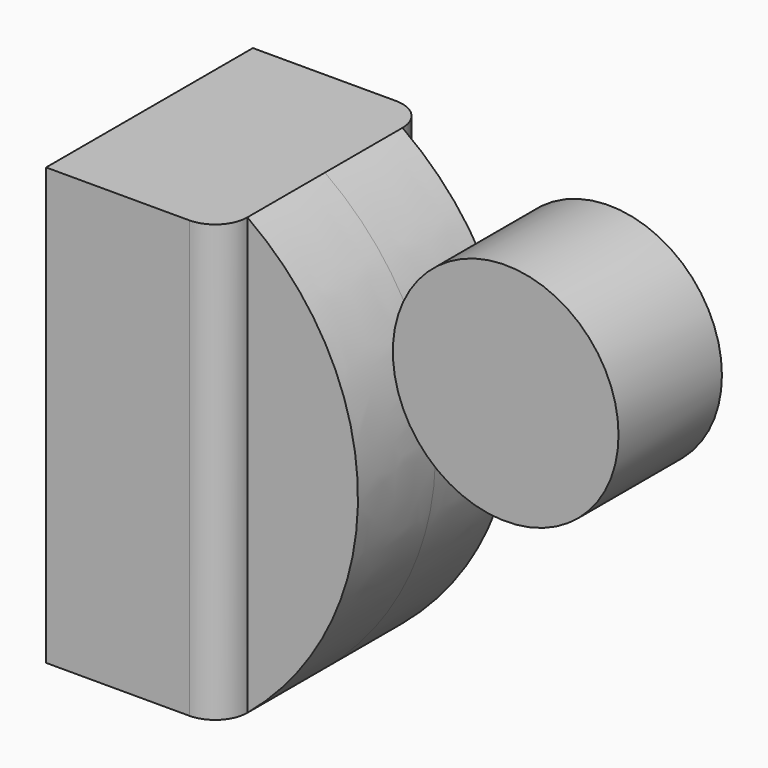
from build123d import *

# Parameters (mm, degrees)
F0_W     = 34.4880186021
F0_H     = 85.7237949967
F1_DEPTH = 25.4
F2_DEPTH = 19.05
F3_R     = 6.34999
F0_R     = 22.1763652159
F0_R_2   = 9.4763652159
F4_DEPTH = 12.7
F5_DEPTH = 12.7
F6_D     = 6.35
F6_DEPTH = 25.401


# Not quite as in the source:
# - a fillet or chamfer is up to 0.001 mm smaller than in the source, because OpenCascade refuses the exact size


with BuildPart() as f1:
    # F0 (on Front) → F1 (new body, symmetric)
    with BuildSketch(Plane.XZ):
        with Locations((-29.842576012, -3.5368986428)):
            Rectangle(F0_W, F0_H)
    extrude(amount=F1_DEPTH, both=True)

    # F0 (on Front) → F2 (join, symmetric)
    with BuildSketch(Plane.XZ):
        with BuildLine():
            Line((-12.5985667109, 39.3249988556), (-12.5985667109, -46.3987961411))
            add(Edge.make_bspline(
                [(-12.5985667109, 39.3249988556), (16.6084952652, 18.4920281172), (16.1393098533, -22.3401486874), (-12.5985667109, -46.3987961411)],
                knots=[0, 0, 0, 0, 85.7237949967, 85.7237949967, 85.7237949967, 85.7237949967], degree=3))
        make_face()
    extrude(amount=F2_DEPTH, both=True)

    # F3 (radius 6.35 in the source; OpenCascade refuses exactly that, so slightly less here)
    f3_edges = [f1.edges().sort_by_distance(p)[0] for p in [
        (-12.598567, -25.4, -3.536899),
        (-12.598567, 25.4, -3.536899),
    ]]
    fillet(f3_edges, radius=F3_R)


with BuildPart() as f4:
    # F0 (on Front) → F4 (new body, symmetric)
    with BuildSketch(Plane.XZ):
        with Locations((33.0783426762, 21.1644805968)):
            Circle(F0_R)
        with Locations((33.0783426762, 21.1644805968)):
            Circle(F0_R_2, mode=Mode.SUBTRACT)
    extrude(amount=F4_DEPTH, both=True)

    # F0 (on Front) → F5 (join, symmetric)
    with BuildSketch(Plane.XZ):
        with Locations((33.0783426762, 21.1644805968)):
            Circle(F0_R_2)
    extrude(amount=F5_DEPTH, both=True)

    # F6 (through all, one way)
    with BuildSketch(Plane.XZ):
        with Locations((33.0783426762, 21.1644805968)):
            Circle(F6_D / 2)
    extrude(amount=-F6_DEPTH, mode=Mode.SUBTRACT)


solid = Compound([f1.part, f4.part])
